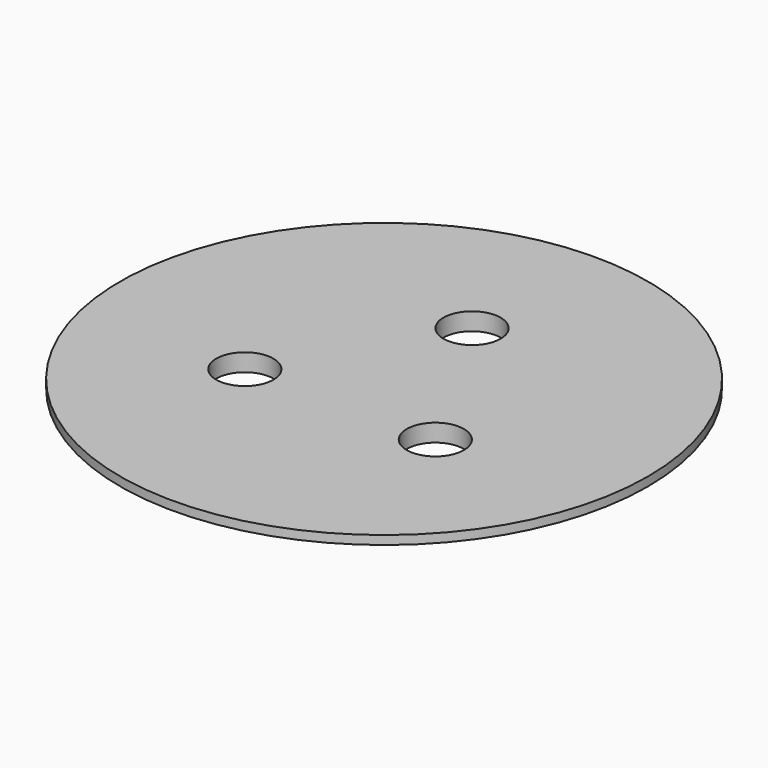
from build123d import *

# Parameters (mm, degrees)
F1_R            = 25
F1_R_2          = 3.25
F2_DEPTH        = 2
F1_R_3          = 30
F3_DEPTH        = 1
F4_DEPTH        = 25
F4_COPIES_COUNT = 3


# Not quite as in the source:
# - a pattern or mirror of a feature is missing from the dataset's text; its kind, count and spacing are read off the source's solid


with BuildPart() as f2:
    # F1 (on Top) → F2 (new body)
    with BuildSketch(Plane.XY):
        Circle(F1_R)
        with Locations((0, 12.5)):
            Circle(F1_R_2, mode=Mode.SUBTRACT)
        with Locations((0, 12.5)):
            Circle(F1_R_2)
    extrude(amount=-F2_DEPTH)

    # F1 (on Top) → F3 (join)
    with BuildSketch(Plane.XY):
        Circle(F1_R_3)
        Circle(F1_R, mode=Mode.SUBTRACT)
    extrude(amount=-F3_DEPTH)

    # F1 (on Top) → F4 (cut)
    with BuildSketch(Plane.XY):
        with Locations((0, 12.5)):
            Circle(F1_R_2)
    f4 = extrude(amount=-F4_DEPTH, mode=Mode.SUBTRACT)

    # F4_copies: F4 ×3 about axis
    f4_copies_axis = Axis((0, 0, 0), (0, 0, 1))
    for i in range(1, F4_COPIES_COUNT):
        add(f4.rotate(f4_copies_axis, i * 360 / F4_COPIES_COUNT), mode=Mode.SUBTRACT)


solid = f2.part
